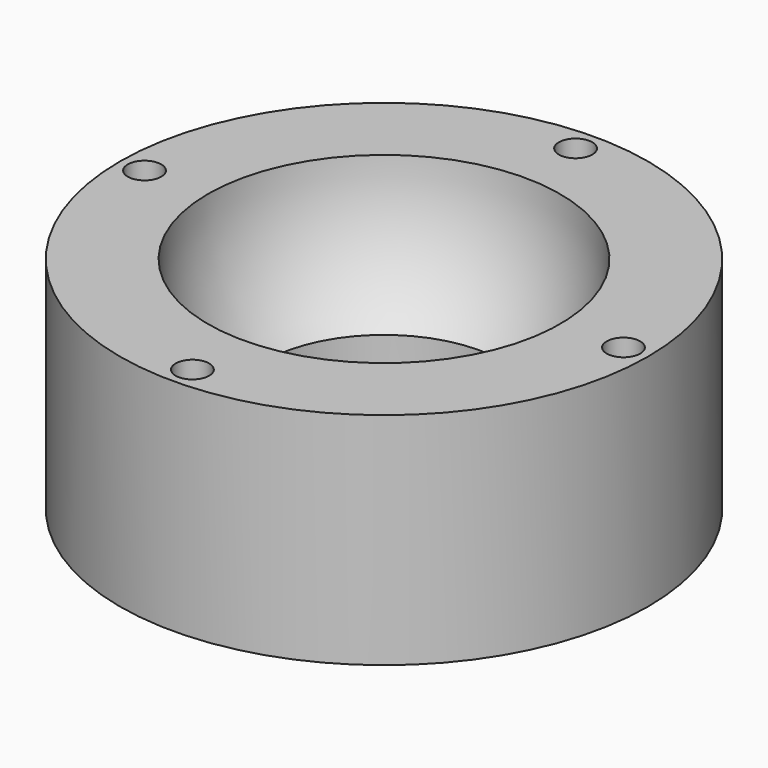
from build123d import *

# Parameters (mm, degrees)
F3_R            = 17.272
F4_DEPTH        = 25.4
F5_SIZE         = 6.35
F7_D            = 4.826
F7_COPIES_COUNT = 4


# Not quite as in the source:
# - a pattern or mirror of a feature is missing from the dataset's text; its kind, count and spacing are read off the source's solid


with BuildPart() as f1:
    # F0 (on Front) → F1 (revolve)
    with BuildSketch(Plane.XZ):
        with BuildLine():
            ThreePointArc((0, -25.4), (-17.9605122421, -17.9605122421), (-25.4, 0))
            Line((-25.4, 0), (-38.1, 0))
            Line((-38.1, 0), (-38.1, -31.75))
            Line((-38.1, -31.75), (0, -31.75))
            Line((0, -31.75), (0, -25.4))
        make_face()
    revolve(axis=Axis((0, 0, -28.575), (0, 0, 1)))

    # F3 (on offset) → F4 (cut)
    with BuildSketch(Plane.XY.offset(-37.2872)):
        Circle(F3_R)
    extrude(amount=F4_DEPTH, mode=Mode.SUBTRACT)

    # F5
    f5_edges = [f1.edges().sort_by_distance(p)[0] for p in [
        (-17.272, 0, -31.75),
    ]]
    chamfer(f5_edges, length=F5_SIZE)

    # F7 (through all)
    with Locations(Plane.XY):
        with Locations((0, -34.544)):
            f7 = Hole(F7_D / 2)

    # F7_copies: F7 ×4 about axis
    f7_copies_axis = Axis((0, 0, 0), (0, 0, 1))
    for i in range(1, F7_COPIES_COUNT):
        add(f7.rotate(f7_copies_axis, i * 360 / F7_COPIES_COUNT), mode=Mode.SUBTRACT)


solid = f1.part
